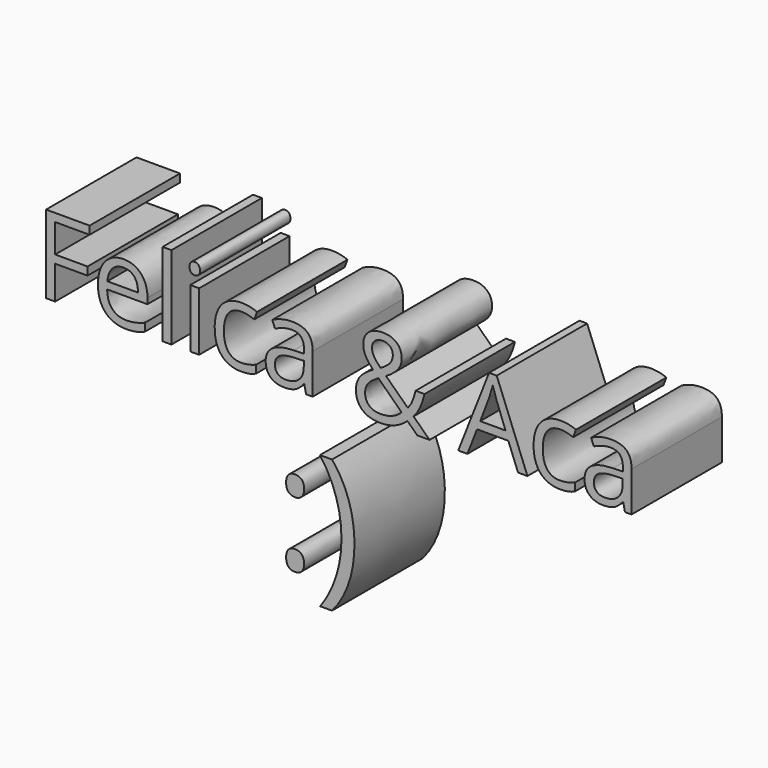
from build123d import *

# Parameters (mm, degrees)
F0_TEXT_SIZE   = 24.5936758195
F0_TEXT_SIZE_2 = 34.2899946392
F1_DEPTH       = 25.4


# Not quite as in the source:
# - Text() gives the source's letters only with a copy of the font that has no kerning and outlines rounded to 1/6400 em; it was checked with that copy


with BuildPart() as f1:
    # F0 (on Front) → F1 (new body)
    with BuildSketch(Plane.XZ):
        with Locations((-73.9536508918, 20.7162927836)):
            Text('Felica & Aca', F0_TEXT_SIZE, font='Open Sans', text_align=(TextAlign.LEFT, TextAlign.BOTTOM))
        with Locations((-20.1239406039, -14.7712612525)):
            Text(':)', F0_TEXT_SIZE_2, font='Open Sans', text_align=(TextAlign.LEFT, TextAlign.BOTTOM))
    extrude(amount=F1_DEPTH)


solid = f1.part
